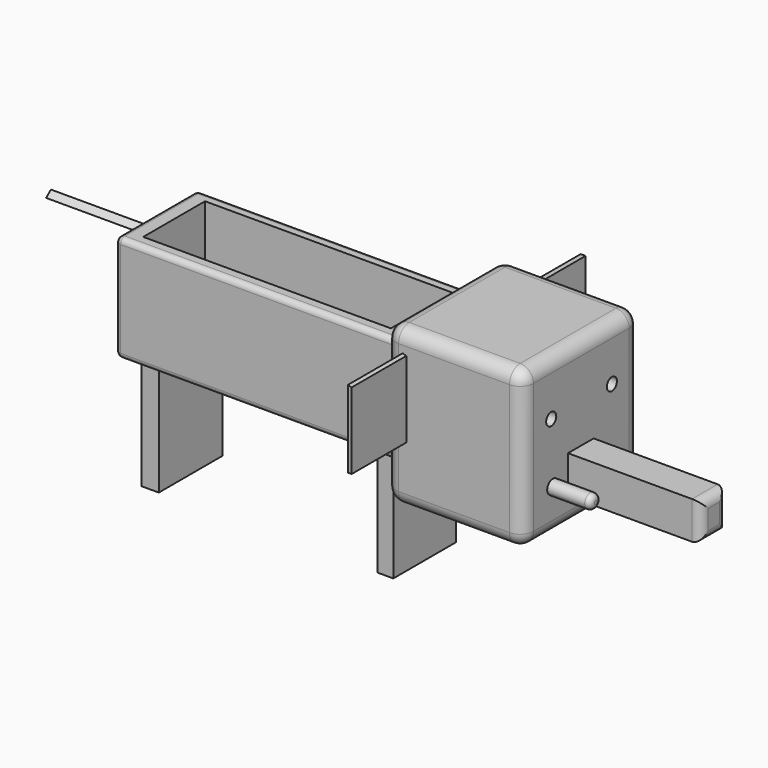
from build123d import *

# Parameters (mm, degrees)
F0_W      = 271.8892842531
F0_H      = 97.4458288401
F1_DEPTH  = 101.6
F3_R      = 5.08
F4_W      = 16.6076868773
F4_H      = 76.0046169162
F5_DEPTH  = 107.696
F6_W      = 15.0446221232
F6_H      = 74.8323127627
F7_DEPTH  = 107.696
F2_W      = 236.4497035742
F2_H      = 73.7357586622
F8_DEPTH  = 77.978
F9_W      = 139.5306698978
F9_H      = 149.727134034
F10_DEPTH = 131.318
F11_R     = 12.7
F12_W     = 30.5456686765
F12_H     = 35.9262302518
F13_DEPTH = 127
F15_DEPTH = 65.278
F17_DEPTH = 70.104
F18_R     = 6.7219361341
F19_DEPTH = 40.894
F21_DEPTH = 100.584
F22_R     = 6.0147460443
F23_DEPTH = 25.4
F24_R     = 5.08
F25_R     = 8.5849434278


with BuildPart() as f1:
    # F0 (on Top) → F1 (new body)
    with BuildSketch(Plane.XY):
        with Locations((10.5727538466, -18.0099094287)):
            Rectangle(F0_W, F0_H)
    extrude(amount=F1_DEPTH)

    # F3
    f3_edges = [f1.edges().sort_by_distance(p)[0] for p in [
        (-125.371888, -66.732824, 50.8),
        (146.517396, -66.732824, 50.8),
        (10.572754, -66.732824, 0),
        (10.572754, -66.732824, 101.6),
        (146.517396, 30.713005, 50.8),
        (146.517396, -18.009909, 0),
        (146.517396, -18.009909, 101.6),
        (-125.371888, 30.713005, 50.8),
        (10.572754, 30.713005, 0),
        (10.572754, 30.713005, 101.6),
        (-125.371888, -18.009909, 0),
        (-125.371888, -18.009909, 101.6),
    ]]
    fillet(f3_edges, radius=F3_R)

    # F4 (on face) → F5 (join)
    with BuildSketch(Plane(origin=(0, 0, 0), x_dir=(1, 0, 0), z_dir=(0, 0, -1))):
        with Locations((-101.2849360704, 17.3892304301)):
            Rectangle(F4_W, F4_H)
    extrude(amount=F5_DEPTH)

    # F6 (on face) → F7 (join)
    with BuildSketch(Plane(origin=(0, 0, 0), x_dir=(1, 0, 0), z_dir=(0, 0, -1))):
        with Locations((122.6258315146, 16.998462379)):
            Rectangle(F6_W, F6_H)
    extrude(amount=F7_DEPTH)

    # F2 (on face) → F8 (cut)
    with BuildSketch(Plane.XY.offset(101.6)):
        with Locations((9.42825526, -17.3080377281)):
            Rectangle(F2_W, F2_H)
    extrude(amount=-F8_DEPTH, mode=Mode.SUBTRACT)

    # F9 (on face) → F10 (join)
    with BuildSketch(Plane.YZ.offset(146.5173959732)):
        with Locations((-14.6516356617, 49.1371015087)):
            Rectangle(F9_W, F9_H)
    extrude(amount=F10_DEPTH)

    # F11
    f11_edges = [f1.edges().sort_by_distance(p)[0] for p in [
        (212.176396, 55.113699, 124.000669),
        (212.176396, -84.416971, 124.000669),
        (146.517396, -14.651636, 124.000669),
        (277.835396, -14.651636, 124.000669),
        (212.176396, -84.416971, -25.726466),
        (146.517396, -84.416971, 49.137102),
        (277.835396, -84.416971, 49.137102),
        (277.835396, -14.651636, -25.726466),
        (277.835396, 55.113699, 49.137102),
        (212.176396, 55.113699, -25.726466),
        (146.517396, 55.113699, 49.137102),
        (146.517396, -14.651636, -25.726466),
    ]]
    fillet(f11_edges, radius=F11_R)

    # F12 (on face) → F13 (join)
    with BuildSketch(Plane.YZ.offset(277.8353959732)):
        with Locations((-15.2728343382, 17.9631151259)):
            Rectangle(F12_W, F12_H)
    extrude(amount=F13_DEPTH)

    # F14 (on face) → F15 (join)
    with BuildSketch(Plane.XZ.offset(84.4169706106)):
        Polygon((166.5966212749, 103.4740507603), (163.0362123251, 104.4450700283), (163.0362123251, 30.6476131082), (166.5966212749, 30.6476131082), align=None)
    extrude(amount=F15_DEPTH)

    # F16 (on face) → F17 (join)
    with BuildSketch(Plane(origin=(0, 55.1136992872, 0), x_dir=(-1, 0, 0), z_dir=(0, 1, 0))):
        Polygon((-165.8086842582, 36.9507782161), (-165.3019338846, 103.3622100949), (-169.9908971786, 103.3622100949), (-169.9908971786, 36.9507782161), align=None)
    extrude(amount=F17_DEPTH)

    # F18 (on face) → F19 (join)
    with BuildSketch(Plane.YZ.offset(277.8353959732)):
        with Locations((-48.636149615, 15.0712924078)):
            Circle(F18_R)
        with Locations((15.748, 15.494)):
            Circle(F18_R)
    extrude(amount=F19_DEPTH)

    # F20 (on face) → F21 (join)
    with BuildSketch(Plane(origin=(-125.3718882799, 0, 0), x_dir=(0, -1, 0), z_dir=(-1, 0, 0))):
        Polygon((23.6901119351, 83.874464035), (17.8975313902, 88.5533466935), (17.8975313902, 83.874464035), align=None)
    extrude(amount=F21_DEPTH)

    # F22 (on face) → F23 (cut)
    with BuildSketch(Plane.YZ.offset(277.8353959732)):
        with Locations((-50.5576916039, 72.7600604296)):
            Circle(F22_R)
        with Locations((21.8323083961, 72.7600604296)):
            Circle(F22_R)
    extrude(amount=-F23_DEPTH, mode=Mode.SUBTRACT)

    # F24
    f24_edges = [f1.edges().sort_by_distance(p)[0] for p in [
        (318.729396, -55.358086, 15.071292),
        (318.729396, 9.026064, 15.494),
    ]]
    fillet(f24_edges, radius=F24_R)

    # F25
    f25_edges = [f1.edges().sort_by_distance(p)[0] for p in [
        (404.835396, -15.272834, 35.92623),
        (404.835396, -30.545669, 17.963115),
        (404.835396, -15.272834, 0),
        (404.835396, 0, 17.963115),
    ]]
    fillet(f25_edges, radius=F25_R)


solid = f1.part
